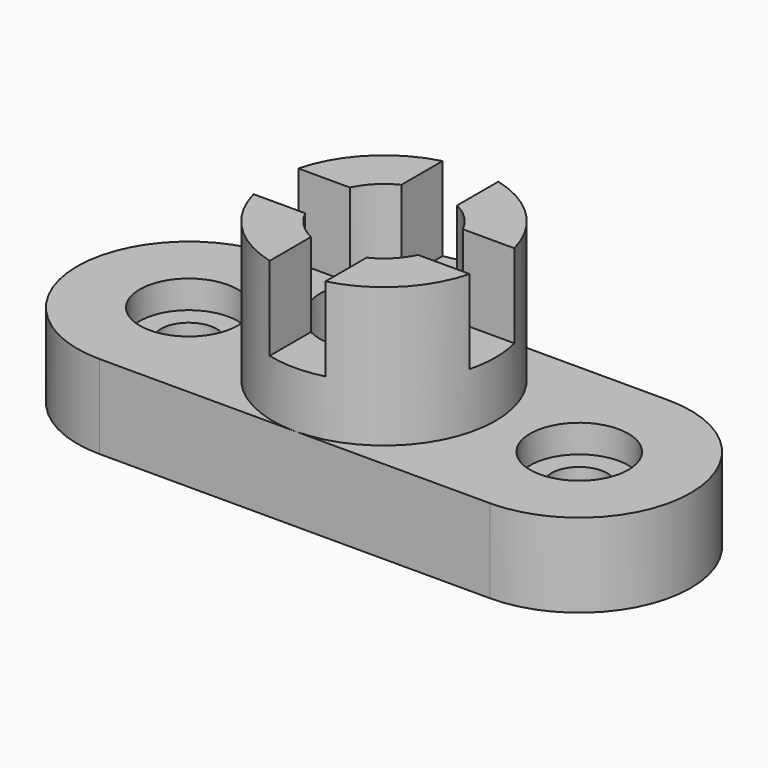
from build123d import *

# Parameters (mm, degrees)
F1_DEPTH  = 19.05
F2_R      = 11.176
F3_DEPTH  = 6.35
F4_R      = 6.35
F5_DEPTH  = 19.051
F6_R      = 25.4
F7_DEPTH  = 31.75
F8_R      = 14.351
F9_DEPTH  = 50.801
F10_W     = 12.7
F10_H     = 12.7
F11_DEPTH = 19.05
F12_DEPTH = 19.05


with BuildPart() as f1:
    # F0 (on Top) → F1 (new body)
    with BuildSketch(Plane.XY):
        with BuildLine():
            Line((44.45, 25.4), (-44.45, 25.4))
            ThreePointArc((-44.45, 25.4), (-69.85, 0), (-44.45, -25.4))
            Line((-44.45, -25.4), (44.45, -25.4))
            ThreePointArc((44.45, -25.4), (69.85, 0), (44.45, 25.4))
        make_face()
    extrude(amount=F1_DEPTH)

    # F2 (on face) → F3 (cut)
    with BuildSketch(Plane.XY.offset(19.05)):
        with Locations((-44.45, 0)):
            Circle(F2_R)
        with Locations((44.45, 0)):
            Circle(F2_R)
    extrude(amount=-F3_DEPTH, mode=Mode.SUBTRACT)

    # F4 (on face) → F5 (cut, through all)
    with BuildSketch(Plane.XY.offset(19.05)):
        with Locations((-44.45, 0)):
            Circle(F4_R)
        with Locations((44.45, 0)):
            Circle(F4_R)
    extrude(amount=-F5_DEPTH, mode=Mode.SUBTRACT)

    # F6 (on face) → F7 (join)
    with BuildSketch(Plane.XY.offset(19.05)):
        Circle(F6_R)
    extrude(amount=F7_DEPTH)

    # F8 (on face) → F9 (cut, through all)
    with BuildSketch(Plane.XY.offset(50.8)):
        Circle(F8_R)
    extrude(amount=-F9_DEPTH, mode=Mode.SUBTRACT)

    # F10 (on face) → F11 (cut)
    with BuildSketch(Plane.XY.offset(50.8)):
        with BuildLine():
            Line((-12.8696814646, 6.35), (-24.5934442484, 6.35))
            ThreePointArc((-24.5934442484, 6.35), (-25.4, 0), (-24.5934442484, -6.35))
            Line((-24.5934442484, -6.35), (-12.8696814646, -6.35))
            ThreePointArc((-12.8696814646, -6.35), (-14.351, 0), (-12.8696814646, 6.35))
        make_face()
        with BuildLine():
            ThreePointArc((6.35, 24.5934442484), (0, 25.4), (-6.35, 24.5934442484))
            Line((-6.35, 24.5934442484), (-6.35, 12.8696814646))
            ThreePointArc((-6.35, 12.8696814646), (0, 14.351), (6.35, 12.8696814646))
            Line((6.35, 12.8696814646), (6.35, 24.5934442484))
        make_face()
        Rectangle(F10_W, F10_H)
        with BuildLine():
            Line((-6.35, -12.8696814646), (-6.35, -24.5934442484))
            ThreePointArc((-6.35, -24.5934442484), (0, -25.4), (6.35, -24.5934442484))
            Line((6.35, -24.5934442484), (6.35, -12.8696814646))
            ThreePointArc((6.35, -12.8696814646), (0, -14.351), (-6.35, -12.8696814646))
        make_face()
        with BuildLine():
            ThreePointArc((25.4, 0), (25.1975542852, 3.2005090291), (24.5934442484, 6.35))
            Line((24.5934442484, 6.35), (12.8696814646, 6.35))
            ThreePointArc((12.8696814646, 6.35), (13.9757647322, 3.260245566), (14.351, 0))
            ThreePointArc((14.351, 0), (13.9757647322, -3.260245566), (12.8696814646, -6.35))
            Line((12.8696814646, -6.35), (24.5934442484, -6.35))
            ThreePointArc((24.5934442484, -6.35), (25.1975542852, -3.2005090291), (25.4, 0))
        make_face()
    extrude(amount=-F11_DEPTH, mode=Mode.SUBTRACT)

    # F10 (on face) → F12 (cut)
    with BuildSketch(Plane.XY.offset(50.8)):
        with BuildLine():
            ThreePointArc((6.35, 24.5934442484), (0, 25.4), (-6.35, 24.5934442484))
            Line((-6.35, 24.5934442484), (-6.35, 12.8696814646))
            ThreePointArc((-6.35, 12.8696814646), (0, 14.351), (6.35, 12.8696814646))
            Line((6.35, 12.8696814646), (6.35, 24.5934442484))
        make_face()
        with BuildLine():
            Line((-6.35, 12.8696814646), (-6.35, 6.35))
            Line((-6.35, 6.35), (6.35, 6.35))
            Line((6.35, 6.35), (6.35, 12.8696814646))
            ThreePointArc((6.35, 12.8696814646), (0, 14.351), (-6.35, 12.8696814646))
        make_face()
        Rectangle(F10_W, F10_H)
        with BuildLine():
            Line((6.35, -6.35), (-6.35, -6.35))
            Line((-6.35, -6.35), (-6.35, -12.8696814646))
            ThreePointArc((-6.35, -12.8696814646), (0, -14.351), (6.35, -12.8696814646))
            Line((6.35, -12.8696814646), (6.35, -6.35))
        make_face()
        with BuildLine():
            Line((-6.35, -12.8696814646), (-6.35, -24.5934442484))
            ThreePointArc((-6.35, -24.5934442484), (0, -25.4), (6.35, -24.5934442484))
            Line((6.35, -24.5934442484), (6.35, -12.8696814646))
            ThreePointArc((6.35, -12.8696814646), (0, -14.351), (-6.35, -12.8696814646))
        make_face()
    extrude(amount=-F12_DEPTH, mode=Mode.SUBTRACT)


solid = f1.part
